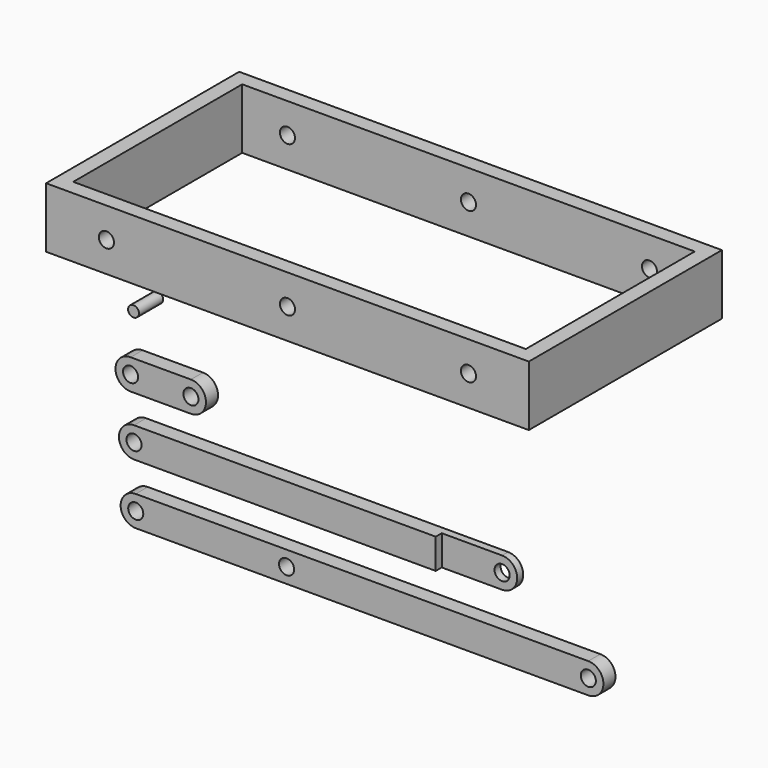
from build123d import *

# Parameters (mm, degrees)
F1_R      = 1.25
F2_DEPTH  = 2.5
F3_R      = 1.25
F4_DEPTH  = 2.5
F5_R      = 1.25
F6_DEPTH  = 2.5
F8_W      = 80
F8_H      = 40
F8_W_2    = 75
F8_H_2    = 35
F9_DEPTH  = 10
F10_R     = 1.25
F11_DEPTH = 40.001
F12_R     = 0.9
F13_DEPTH = 5
F15_DEPTH = 1.25


with BuildPart() as f2:
    # F1 (on Front) → F2 (new body)
    with BuildSketch(Plane.XZ):
        with BuildLine():
            Line((10, 2.5), (0, 2.5))
            ThreePointArc((0, 2.5), (-2.5, 0), (0, -2.5))
            Line((0, -2.5), (10, -2.5))
            ThreePointArc((10, -2.5), (12.5, 0), (10, 2.5))
        make_face()
        Circle(F1_R, mode=Mode.SUBTRACT)
        with Locations((10, 0)):
            Circle(F1_R, mode=Mode.SUBTRACT)
    extrude(amount=F2_DEPTH)


with BuildPart() as f4:
    # F3 (on Front) → F4 (new body)
    with BuildSketch(Plane.XZ):
        with BuildLine():
            Line((60.5706622079, -7.232673876), (0.5706622079, -7.232673876))
            ThreePointArc((0.5706622079, -7.232673876), (-1.9293377921, -9.732673876), (0.5706622079, -12.232673876))
            Line((0.5706622079, -12.232673876), (60.5706622079, -12.232673876))
            ThreePointArc((60.5706622079, -12.232673876), (63.0706622079, -9.732673876), (60.5706622079, -7.232673876))
        make_face()
        with Locations((0.5706622079, -9.732673876)):
            Circle(F3_R, mode=Mode.SUBTRACT)
        with Locations((60.5706622079, -9.732673876)):
            Circle(F3_R, mode=Mode.SUBTRACT)
    extrude(amount=F4_DEPTH)

    # F14 (on face) → F15 (cut)
    with BuildSketch(Plane.XZ.offset(2.5)):
        with BuildLine():
            Line((50.5706622079, -12.232673876), (60.5706622079, -12.232673876))
            ThreePointArc((60.5706622079, -12.232673876), (63.0706622079, -9.732673876), (60.5706622079, -7.232673876))
            Line((60.5706622079, -7.232673876), (50.5706622079, -7.232673876))
            Line((50.5706622079, -7.232673876), (50.5706622079, -12.232673876))
        make_face()
    extrude(amount=-F15_DEPTH, mode=Mode.SUBTRACT)


with BuildPart() as f6:
    # F5 (on Front) → F6 (new body)
    with BuildSketch(Plane.XZ):
        with BuildLine():
            Line((75.8570737601, -17.1626018733), (0.8570737601, -17.1626018733))
            ThreePointArc((0.8570737601, -17.1626018733), (-1.6429262399, -19.6626018733), (0.8570737601, -22.1626018733))
            Line((0.8570737601, -22.1626018733), (75.8570737601, -22.1626018733))
            ThreePointArc((75.8570737601, -22.1626018733), (78.3570737601, -19.6626018733), (75.8570737601, -17.1626018733))
        make_face()
        with Locations((0.8570737601, -19.6626018733)):
            Circle(F5_R, mode=Mode.SUBTRACT)
        with Locations((25.8570737601, -19.6626018733)):
            Circle(F5_R, mode=Mode.SUBTRACT)
        with Locations((75.8570737601, -19.6626018733)):
            Circle(F5_R, mode=Mode.SUBTRACT)
    extrude(amount=F6_DEPTH)


with BuildPart() as f9:
    # F8 (on offset) → F9 (new body)
    with BuildSketch(Plane.XY.offset(25)):
        with Locations((40, 0)):
            Rectangle(F8_W, F8_H)
        with Locations((40, 0)):
            Rectangle(F8_W_2, F8_H_2, mode=Mode.SUBTRACT)
    extrude(amount=F9_DEPTH)

    # F10 (on face) → F11 (cut, through all)
    with BuildSketch(Plane.XZ.offset(20)):
        with Locations((10, 30)):
            Circle(F10_R)
        with Locations((70, 30)):
            Circle(F10_R)
        with Locations((40, 30)):
            Circle(F10_R)
    extrude(amount=-F11_DEPTH, mode=Mode.SUBTRACT)


with BuildPart() as f13:
    # F12 (on Front) → F13 (new body)
    with BuildSketch(Plane.XZ):
        with Locations((2.488047583, 11.0218990594)):
            Circle(F12_R)
    extrude(amount=F13_DEPTH)


solid = Compound([f2.part, f4.part, f6.part, f9.part, f13.part])
